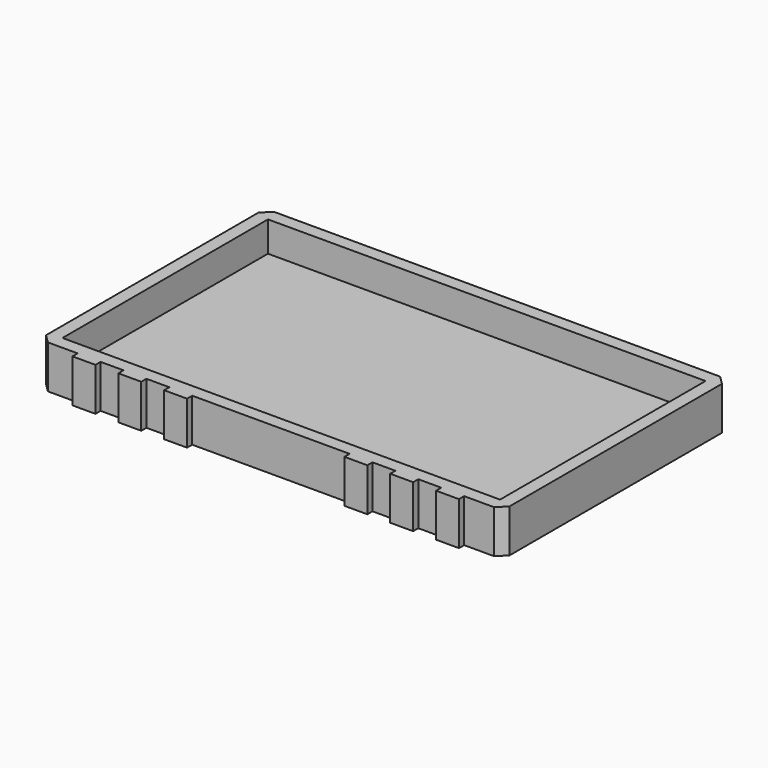
from build123d import *

# Parameters (mm, degrees)
F1_DEPTH = 5
F2_T     = -3
F3_SIZE  = 2
F4_W     = 5.3098537028
F4_H     = 10
F5_DEPTH = 1.5


# Not quite as in the source:
# - a pattern or mirror of a feature is missing from the dataset's text; its kind, count and spacing are read off the source's solid


with BuildPart() as f1:
    # F0 (on Top) → F1 (new body, symmetric)
    with BuildSketch(Plane.XY):
        Polygon((53.696885705, 32.7549055219), (0, 32.7549055219), (-53.696885705, 32.7549055219), (-53.696885705, 0), (-53.696885705, -32.7549055219), (0, -32.7549055219), (53.696885705, -32.7549055219), (53.696885705, 0), align=None)
    extrude(amount=F1_DEPTH, both=True)

    # F2
    f2_openings = [f1.faces().sort_by_distance(p)[0] for p in [
        (0, 0, 5),
    ]]
    offset(amount=F2_T, openings=f2_openings)

    # F3
    f3_edges = [f1.edges().sort_by_distance(p)[0] for p in [
        (53.696886, -32.754906, 0),
        (-53.696886, 32.754906, 0),
        (53.696886, 32.754906, 0),
        (-53.696886, -32.754906, 0),
    ]]
    chamfer(f3_edges, length=F3_SIZE)

    # F4 (on face) → F5 (join)
    with BuildSketch(Plane.XZ.offset(32.7549055219)):
        with Locations((-42.1222578734, 0)):
            Rectangle(F4_W, F4_H)
        with Locations((-31.5025504678, 0)):
            Rectangle(F4_W, F4_H)
        with Locations((-20.8828430623, 0)):
            Rectangle(F4_W, F4_H)
    f5 = extrude(amount=F5_DEPTH)

    # F5_copies: F5 across plane
    add(f5.mirror(Plane(origin=(0, 0, 0), x_dir=(0, 0, 1), z_dir=(1, 0, 0))))


solid = f1.part
